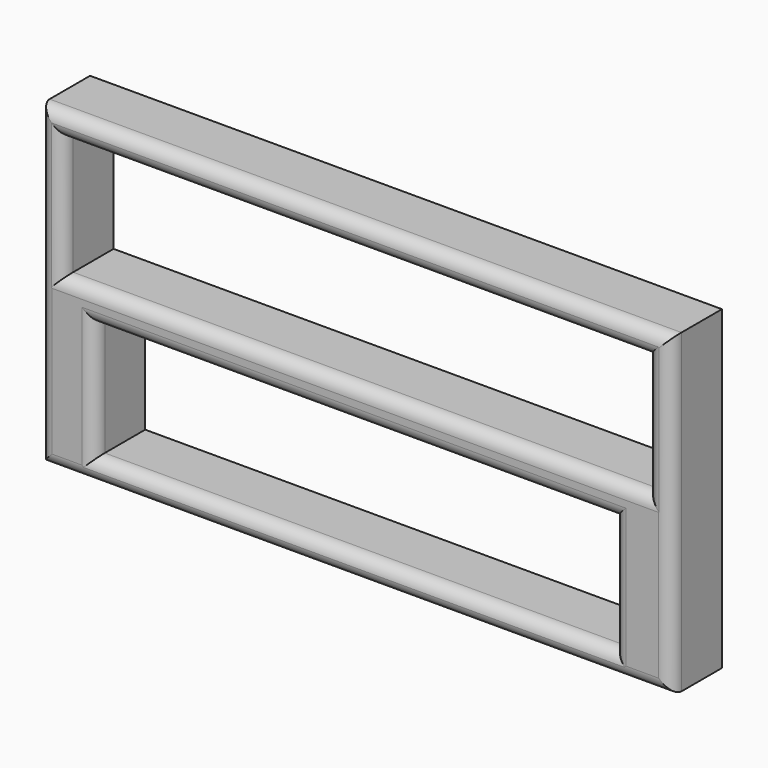
from build123d import *

# Parameters (mm, degrees)
F0_W         = 254
F0_H         = 127
F2_DEPTH     = 25.4
F1_W         = 234.5826178789
F1_H         = 48.6704111099
F1_W_2       = 208.4935232997
F1_H_2       = 46.9165234827
F3_DEPTH     = 50.8
F4_DEPTH     = 102.87
F5_T1_DEPTH  = 279.4
F5_T3_DEPTH  = 152.4
F5_T5_DEPTH  = 46.9165234827
F5_T7_DEPTH  = 208.4935232997
F5_T9_DEPTH  = 48.6704111099
F5_T11_DEPTH = 234.5826178789
F5_T17_DEPTH = 59.6165234827
F5_T21_DEPTH = 221.1935232997
F5_T28_DEPTH = 59.6165234827
F5_T32_DEPTH = 221.1935232997
F5_T39_DEPTH = 221.1935232997
F5_T43_DEPTH = 59.6165234827
F5_T50_DEPTH = 59.6165234827
F5_T54_DEPTH = 221.1935232997
F5_T61_DEPTH = 61.3704111099
F5_T65_DEPTH = 247.2826178789
F5_T72_DEPTH = 61.3704111099
F5_T76_DEPTH = 247.2826178789
F5_T83_DEPTH = 247.2826178789
F5_T87_DEPTH = 61.3704111099
F5_T94_DEPTH = 61.3704111099
F5_T98_DEPTH = 247.2826178789


# Not quite as in the source:
# - a fillet or chamfer that OpenCascade refuses, or shapes differently, is made with other operations: its cross-section is extruded or revolved along the edge and cut away or added


with BuildPart() as f2:
    # F0 (on Front) → F2 (new body)
    with BuildSketch(Plane.XZ):
        Rectangle(F0_W, F0_H)
    extrude(amount=F2_DEPTH)

    # F1 (on face) → F3 (cut)
    with BuildSketch(Plane.XZ):
        with Locations((-0.2548918128, 29.650695622)):
            Rectangle(F1_W, F1_H)
        with Locations((-0.5837492645, -31.0777008999)):
            Rectangle(F1_W_2, F1_H_2)
    extrude(amount=-F3_DEPTH, mode=Mode.SUBTRACT)

    # F1 (on face) → F4 (cut)
    with BuildSketch(Plane.XZ):
        with Locations((-0.2548918128, 29.650695622)):
            Rectangle(F1_W, F1_H)
        with Locations((-0.5837492645, -31.0777008999)):
            Rectangle(F1_W_2, F1_H_2)
    extrude(amount=F4_DEPTH, mode=Mode.SUBTRACT)

    # F5: fillet of radius 5.08 on 12 edges, made by hand

    # F5_s2 → F5_t1 (cut)
    with BuildSketch(Plane.YZ.offset(-139.7)):
        with BuildLine():
            ThreePointArc((-20.32, -63.5), (-23.9121024484, -62.0121024484), (-25.4, -58.42))
            Line((-25.4, -58.42), (-25.4, -63.5))
            Line((-25.4, -63.5), (-20.32, -63.5))
        make_face()
        with BuildLine():
            ThreePointArc((-25.4, 58.42), (-23.9121024484, 62.0121024484), (-20.32, 63.5))
            Line((-20.32, 63.5), (-25.4, 63.5))
            Line((-25.4, 63.5), (-25.4, 58.42))
        make_face()
    extrude(amount=F5_T1_DEPTH, mode=Mode.SUBTRACT)

    # F5_s4 → F5_t3 (cut)
    with BuildSketch(Plane.XY.offset(-76.2)):
        with BuildLine():
            ThreePointArc((-127, -20.32), (-125.5121024484, -23.9121024484), (-121.92, -25.4))
            Line((-121.92, -25.4), (-127, -25.4))
            Line((-127, -25.4), (-127, -20.32))
        make_face()
        with BuildLine():
            ThreePointArc((127, -20.32), (125.5121024484, -23.9121024484), (121.92, -25.4))
            Line((121.92, -25.4), (127, -25.4))
            Line((127, -25.4), (127, -20.32))
        make_face()
    extrude(amount=F5_T3_DEPTH, mode=Mode.SUBTRACT)

    # F5_s6 → F5_t5 (cut)
    with BuildSketch(Plane.XY.offset(-54.5359626412)):
        with BuildLine():
            ThreePointArc((-109.9105109143, -25.4), (-106.3184084659, -23.9121024484), (-104.8305109143, -20.32))
            Line((-104.8305109143, -20.32), (-104.8305109143, -25.4))
            Line((-104.8305109143, -25.4), (-109.9105109143, -25.4))
        make_face()
        with BuildLine():
            ThreePointArc((108.7430123854, -25.4), (105.1509099369, -23.9121024484), (103.6630123854, -20.32))
            Line((103.6630123854, -20.32), (103.6630123854, -25.4))
            Line((103.6630123854, -25.4), (108.7430123854, -25.4))
        make_face()
    extrude(amount=F5_T5_DEPTH, mode=Mode.SUBTRACT)

    # F5_s8 → F5_t7 (cut)
    with BuildSketch(Plane.YZ.offset(-104.8305109143)):
        with BuildLine():
            ThreePointArc((-25.4, -59.6159626412), (-23.9121024484, -56.0238601928), (-20.32, -54.5359626412))
            Line((-20.32, -54.5359626412), (-25.4, -54.5359626412))
            Line((-25.4, -54.5359626412), (-25.4, -59.6159626412))
        make_face()
        with BuildLine():
            ThreePointArc((-25.4, -2.5394391586), (-23.9121024484, -6.131541607), (-20.32, -7.6194391586))
            Line((-20.32, -7.6194391586), (-25.4, -7.6194391586))
            Line((-25.4, -7.6194391586), (-25.4, -2.5394391586))
        make_face()
    extrude(amount=F5_T7_DEPTH, mode=Mode.SUBTRACT)

    # F5_s10 → F5_t9 (cut)
    with BuildSketch(Plane.XY.offset(5.315490067)):
        with BuildLine():
            ThreePointArc((-122.6262007523, -25.4), (-119.0340983038, -23.9121024484), (-117.5462007523, -20.32))
            Line((-117.5462007523, -20.32), (-117.5462007523, -25.4))
            Line((-117.5462007523, -25.4), (-122.6262007523, -25.4))
        make_face()
        with BuildLine():
            ThreePointArc((122.1164171267, -25.4), (118.5243146782, -23.9121024484), (117.0364171267, -20.32))
            Line((117.0364171267, -20.32), (117.0364171267, -25.4))
            Line((117.0364171267, -25.4), (122.1164171267, -25.4))
        make_face()
    extrude(amount=F5_T9_DEPTH, mode=Mode.SUBTRACT)

    # F5_s12 → F5_t11 (cut)
    with BuildSketch(Plane.YZ.offset(-117.5462007523)):
        with BuildLine():
            ThreePointArc((-25.4, 0.235490067), (-23.9121024484, 3.8275925154), (-20.32, 5.315490067))
            Line((-20.32, 5.315490067), (-25.4, 5.315490067))
            Line((-25.4, 5.315490067), (-25.4, 0.235490067))
        make_face()
        with BuildLine():
            ThreePointArc((-25.4, 59.0659011769), (-23.9121024484, 55.4737987285), (-20.32, 53.9859011769))
            Line((-20.32, 53.9859011769), (-25.4, 53.9859011769))
            Line((-25.4, 53.9859011769), (-25.4, 59.0659011769))
        make_face()
    extrude(amount=F5_T11_DEPTH, mode=Mode.SUBTRACT)


with BuildPart() as f5_tool15:
    # F5_s16 → F5_t17 (new body)
    with BuildSketch(Plane.XY.offset(-67.2359626412)):
        with BuildLine():
            ThreePointArc((-109.9105109143, -25.4), (-106.3184084659, -23.9121024484), (-104.8305109143, -20.32))
            Line((-104.8305109143, -20.32), (-104.8305109143, -25.4))
            Line((-104.8305109143, -25.4), (-109.9105109143, -25.4))
        make_face()
    extrude(amount=F5_T17_DEPTH)

    split(bisect_by=Plane.XY.offset(-54.5359626412), keep=Keep.BOTTOM)


with BuildPart() as f5_tool19:
    # F5_s20 → F5_t21 (new body)
    with BuildSketch(Plane.YZ.offset(103.6630123854)):
        with BuildLine():
            ThreePointArc((-25.4, -59.6159626412), (-23.9121024484, -56.0238601928), (-20.32, -54.5359626412))
            Line((-20.32, -54.5359626412), (-25.4, -54.5359626412))
            Line((-25.4, -54.5359626412), (-25.4, -59.6159626412))
        make_face()
    extrude(amount=-F5_T21_DEPTH)

    split(bisect_by=Plane.YZ.offset(-104.8305109143), keep=Keep.BOTTOM)


with BuildPart() as f5_tool15_1:
    add(f5_tool15.part)

    # F5_t23: intersect F5_tool19
    add(f5_tool19.part, mode=Mode.INTERSECT)


with BuildPart() as f2_1:
    add(f2.part)

    # F5_t13: cut F5_tool15
    add(f5_tool15_1.part, mode=Mode.SUBTRACT)


with BuildPart() as f5_tool26:
    # F5_s27 → F5_t28 (new body)
    with BuildSketch(Plane.XY.offset(-54.5359626412)):
        with BuildLine():
            ThreePointArc((-109.9105109143, -25.4), (-106.3184084659, -23.9121024484), (-104.8305109143, -20.32))
            Line((-104.8305109143, -20.32), (-104.8305109143, -25.4))
            Line((-104.8305109143, -25.4), (-109.9105109143, -25.4))
        make_face()
    extrude(amount=F5_T28_DEPTH)

    split(bisect_by=Plane.XY.offset(-7.6194391586), keep=Keep.TOP)


with BuildPart() as f5_tool30:
    # F5_s31 → F5_t32 (new body)
    with BuildSketch(Plane.YZ.offset(-117.5305109143)):
        with BuildLine():
            ThreePointArc((-25.4, -2.5394391586), (-23.9121024484, -6.131541607), (-20.32, -7.6194391586))
            Line((-20.32, -7.6194391586), (-25.4, -7.6194391586))
            Line((-25.4, -7.6194391586), (-25.4, -2.5394391586))
        make_face()
    extrude(amount=F5_T32_DEPTH)

    split(bisect_by=Plane.YZ.offset(-104.8305109143), keep=Keep.BOTTOM)


with BuildPart() as f5_tool26_1:
    add(f5_tool26.part)

    # F5_t34: intersect F5_tool30
    add(f5_tool30.part, mode=Mode.INTERSECT)


with BuildPart() as f2_2:
    add(f2_1.part)

    # F5_t24: cut F5_tool26
    add(f5_tool26_1.part, mode=Mode.SUBTRACT)


with BuildPart() as f5_tool37:
    # F5_s38 → F5_t39 (new body)
    with BuildSketch(Plane.YZ.offset(116.3630123854)):
        with BuildLine():
            ThreePointArc((-25.4, -59.6159626412), (-23.9121024484, -56.0238601928), (-20.32, -54.5359626412))
            Line((-20.32, -54.5359626412), (-25.4, -54.5359626412))
            Line((-25.4, -54.5359626412), (-25.4, -59.6159626412))
        make_face()
    extrude(amount=-F5_T39_DEPTH)

    split(bisect_by=Plane.YZ.offset(103.6630123854), keep=Keep.TOP)


with BuildPart() as f5_tool41:
    # F5_s42 → F5_t43 (new body)
    with BuildSketch(Plane.XY.offset(-7.6194391586)):
        with BuildLine():
            ThreePointArc((108.7430123854, -25.4), (105.1509099369, -23.9121024484), (103.6630123854, -20.32))
            Line((103.6630123854, -20.32), (103.6630123854, -25.4))
            Line((103.6630123854, -25.4), (108.7430123854, -25.4))
        make_face()
    extrude(amount=-F5_T43_DEPTH)

    split(bisect_by=Plane.XY.offset(-54.5359626412), keep=Keep.BOTTOM)


with BuildPart() as f5_tool37_1:
    add(f5_tool37.part)

    # F5_t45: intersect F5_tool41
    add(f5_tool41.part, mode=Mode.INTERSECT)


with BuildPart() as f2_3:
    add(f2_2.part)

    # F5_t35: cut F5_tool37
    add(f5_tool37_1.part, mode=Mode.SUBTRACT)


with BuildPart() as f5_tool48:
    # F5_s49 → F5_t50 (new body)
    with BuildSketch(Plane.XY.offset(5.0805608414)):
        with BuildLine():
            ThreePointArc((108.7430123854, -25.4), (105.1509099369, -23.9121024484), (103.6630123854, -20.32))
            Line((103.6630123854, -20.32), (103.6630123854, -25.4))
            Line((103.6630123854, -25.4), (108.7430123854, -25.4))
        make_face()
    extrude(amount=-F5_T50_DEPTH)

    split(bisect_by=Plane.XY.offset(-7.6194391586), keep=Keep.TOP)


with BuildPart() as f5_tool52:
    # F5_s53 → F5_t54 (new body)
    with BuildSketch(Plane.YZ.offset(-104.8305109143)):
        with BuildLine():
            ThreePointArc((-25.4, -2.5394391586), (-23.9121024484, -6.131541607), (-20.32, -7.6194391586))
            Line((-20.32, -7.6194391586), (-25.4, -7.6194391586))
            Line((-25.4, -7.6194391586), (-25.4, -2.5394391586))
        make_face()
    extrude(amount=F5_T54_DEPTH)

    split(bisect_by=Plane.YZ.offset(103.6630123854), keep=Keep.TOP)


with BuildPart() as f5_tool48_1:
    add(f5_tool48.part)

    # F5_t56: intersect F5_tool52
    add(f5_tool52.part, mode=Mode.INTERSECT)


with BuildPart() as f2_4:
    add(f2_3.part)

    # F5_t46: cut F5_tool48
    add(f5_tool48_1.part, mode=Mode.SUBTRACT)


with BuildPart() as f5_tool59:
    # F5_s60 → F5_t61 (new body)
    with BuildSketch(Plane.XY.offset(-7.384509933)):
        with BuildLine():
            ThreePointArc((-122.6262007523, -25.4), (-119.0340983038, -23.9121024484), (-117.5462007523, -20.32))
            Line((-117.5462007523, -20.32), (-117.5462007523, -25.4))
            Line((-117.5462007523, -25.4), (-122.6262007523, -25.4))
        make_face()
    extrude(amount=F5_T61_DEPTH)

    split(bisect_by=Plane.XY.offset(5.315490067), keep=Keep.BOTTOM)


with BuildPart() as f5_tool63:
    # F5_s64 → F5_t65 (new body)
    with BuildSketch(Plane.YZ.offset(117.0364171267)):
        with BuildLine():
            ThreePointArc((-25.4, 0.235490067), (-23.9121024484, 3.8275925154), (-20.32, 5.315490067))
            Line((-20.32, 5.315490067), (-25.4, 5.315490067))
            Line((-25.4, 5.315490067), (-25.4, 0.235490067))
        make_face()
    extrude(amount=-F5_T65_DEPTH)

    split(bisect_by=Plane.YZ.offset(-117.5462007523), keep=Keep.BOTTOM)


with BuildPart() as f5_tool59_1:
    add(f5_tool59.part)

    # F5_t67: intersect F5_tool63
    add(f5_tool63.part, mode=Mode.INTERSECT)


with BuildPart() as f2_5:
    add(f2_4.part)

    # F5_t57: cut F5_tool59
    add(f5_tool59_1.part, mode=Mode.SUBTRACT)


with BuildPart() as f5_tool70:
    # F5_s71 → F5_t72 (new body)
    with BuildSketch(Plane.XY.offset(5.315490067)):
        with BuildLine():
            ThreePointArc((-122.6262007523, -25.4), (-119.0340983038, -23.9121024484), (-117.5462007523, -20.32))
            Line((-117.5462007523, -20.32), (-117.5462007523, -25.4))
            Line((-117.5462007523, -25.4), (-122.6262007523, -25.4))
        make_face()
    extrude(amount=F5_T72_DEPTH)

    split(bisect_by=Plane.XY.offset(53.9859011769), keep=Keep.TOP)


with BuildPart() as f5_tool74:
    # F5_s75 → F5_t76 (new body)
    with BuildSketch(Plane.YZ.offset(-130.2462007523)):
        with BuildLine():
            ThreePointArc((-25.4, 59.0659011769), (-23.9121024484, 55.4737987285), (-20.32, 53.9859011769))
            Line((-20.32, 53.9859011769), (-25.4, 53.9859011769))
            Line((-25.4, 53.9859011769), (-25.4, 59.0659011769))
        make_face()
    extrude(amount=F5_T76_DEPTH)

    split(bisect_by=Plane.YZ.offset(-117.5462007523), keep=Keep.BOTTOM)


with BuildPart() as f5_tool70_1:
    add(f5_tool70.part)

    # F5_t78: intersect F5_tool74
    add(f5_tool74.part, mode=Mode.INTERSECT)


with BuildPart() as f2_6:
    add(f2_5.part)

    # F5_t68: cut F5_tool70
    add(f5_tool70_1.part, mode=Mode.SUBTRACT)


with BuildPart() as f5_tool81:
    # F5_s82 → F5_t83 (new body)
    with BuildSketch(Plane.YZ.offset(129.7364171267)):
        with BuildLine():
            ThreePointArc((-25.4, 0.235490067), (-23.9121024484, 3.8275925154), (-20.32, 5.315490067))
            Line((-20.32, 5.315490067), (-25.4, 5.315490067))
            Line((-25.4, 5.315490067), (-25.4, 0.235490067))
        make_face()
    extrude(amount=-F5_T83_DEPTH)

    split(bisect_by=Plane.YZ.offset(117.0364171267), keep=Keep.TOP)


with BuildPart() as f5_tool85:
    # F5_s86 → F5_t87 (new body)
    with BuildSketch(Plane.XY.offset(53.9859011769)):
        with BuildLine():
            ThreePointArc((122.1164171267, -25.4), (118.5243146782, -23.9121024484), (117.0364171267, -20.32))
            Line((117.0364171267, -20.32), (117.0364171267, -25.4))
            Line((117.0364171267, -25.4), (122.1164171267, -25.4))
        make_face()
    extrude(amount=-F5_T87_DEPTH)

    split(bisect_by=Plane.XY.offset(5.315490067), keep=Keep.BOTTOM)


with BuildPart() as f5_tool81_1:
    add(f5_tool81.part)

    # F5_t89: intersect F5_tool85
    add(f5_tool85.part, mode=Mode.INTERSECT)


with BuildPart() as f2_7:
    add(f2_6.part)

    # F5_t79: cut F5_tool81
    add(f5_tool81_1.part, mode=Mode.SUBTRACT)


with BuildPart() as f5_tool92:
    # F5_s93 → F5_t94 (new body)
    with BuildSketch(Plane.XY.offset(66.6859011769)):
        with BuildLine():
            ThreePointArc((122.1164171267, -25.4), (118.5243146782, -23.9121024484), (117.0364171267, -20.32))
            Line((117.0364171267, -20.32), (117.0364171267, -25.4))
            Line((117.0364171267, -25.4), (122.1164171267, -25.4))
        make_face()
    extrude(amount=-F5_T94_DEPTH)

    split(bisect_by=Plane.XY.offset(53.9859011769), keep=Keep.TOP)


with BuildPart() as f5_tool96:
    # F5_s97 → F5_t98 (new body)
    with BuildSketch(Plane.YZ.offset(-117.5462007523)):
        with BuildLine():
            ThreePointArc((-25.4, 59.0659011769), (-23.9121024484, 55.4737987285), (-20.32, 53.9859011769))
            Line((-20.32, 53.9859011769), (-25.4, 53.9859011769))
            Line((-25.4, 53.9859011769), (-25.4, 59.0659011769))
        make_face()
    extrude(amount=F5_T98_DEPTH)

    split(bisect_by=Plane.YZ.offset(117.0364171267), keep=Keep.TOP)


with BuildPart() as f5_tool92_1:
    add(f5_tool92.part)

    # F5_t100: intersect F5_tool96
    add(f5_tool96.part, mode=Mode.INTERSECT)


with BuildPart() as f2_8:
    add(f2_7.part)

    # F5_t90: cut F5_tool92
    add(f5_tool92_1.part, mode=Mode.SUBTRACT)


solid = f2_8.part
